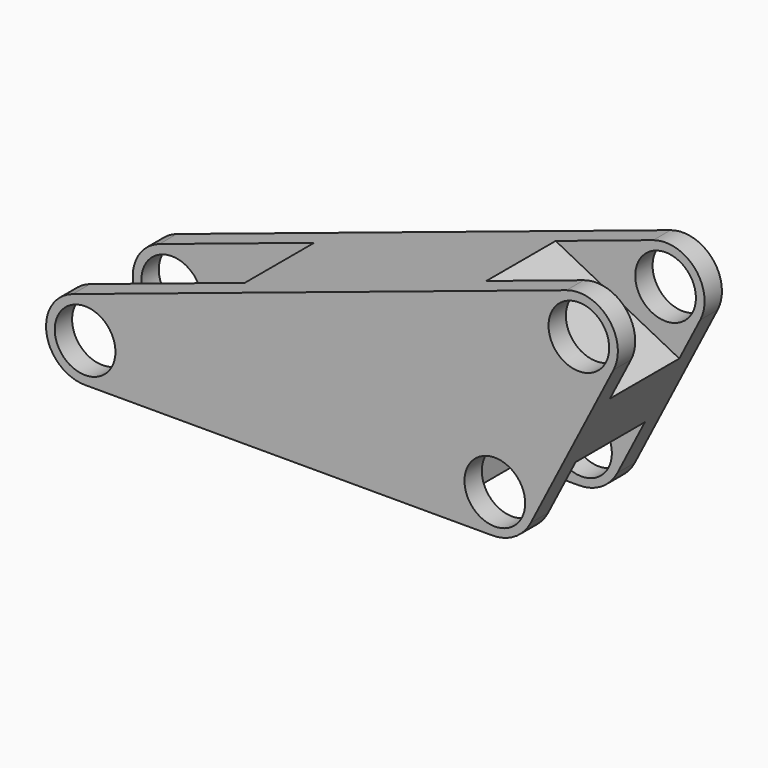
from build123d import *

# Parameters (mm, degrees)
F0_R        = 3.5
F1_DEPTH    = 7.5
F2_W        = 10
F2_H        = 10
F3_DEPTH    = 10
F4_W        = 10
F4_H        = 10
F5_DEPTH    = 10
F6_T1_DEPTH = 10
F7_W        = 10
F7_H        = 14.69305549
F8_DEPTH    = 17.6
F9_DEPTH    = 10
F10_W       = 10
F10_H       = 10
F11_DEPTH   = 25
F12_R       = 5


# Not quite as in the source:
# - a fillet or chamfer that OpenCascade refuses, or shapes differently, is made with other operations: its cross-section is extruded or revolved along the edge and cut away or added
# - a feature of the source that left no trace in its solid (it failed there, or was rolled back) is left out


with BuildPart() as f1:
    # F0 (on Front) → F1 (new body, symmetric)
    with BuildSketch(Plane.XZ):
        with BuildLine():
            ThreePointArc((-12.7951829484, 8.7706469828), (-15.8191748578, 3.7816377734), (-11.3768831394, 0))
            Line((-11.3768831394, 0), (38.6231168606, 0))
            Line((38.6231168606, 0), (49.5697341402, 21.3581733801))
            ThreePointArc((49.5697341402, 21.3581733801), (48.9808970603, 26.3401983487), (44.1467768224, 27.6813111028))
            Line((44.1467768224, 27.6813111028), (-12.7951829484, 8.7706469828))
        make_face()
        with Locations((-11.3768831394, 4.5)):
            Circle(F0_R, mode=Mode.SUBTRACT)
        with Locations((35.8728712662, 4.5)):
            Circle(F0_R, mode=Mode.SUBTRACT)
        with Locations((45.5650766314, 23.41066412)):
            Circle(F0_R, mode=Mode.SUBTRACT)
    extrude(amount=F1_DEPTH, both=True)

    # F2 (on face) → F3 (cut)
    with BuildSketch(Plane(origin=(30.5881386489, 0, -15.6772136421), x_dir=(0, 1, 0), z_dir=(0.8899238908, 0, -0.4561090533))):
        with Locations((0, 22.6163532674)):
            Rectangle(F2_W, F2_H)
    extrude(amount=-F3_DEPTH, mode=Mode.SUBTRACT)

    # F4 (on face) → F5 (cut)
    with BuildSketch(Plane(origin=(0, 0, 0), x_dir=(1, 0, 0), z_dir=(0, 0, -1))):
        with Locations((33.6231168606, 0)):
            Rectangle(F4_W, F4_H)
    extrude(amount=-F5_DEPTH, mode=Mode.SUBTRACT)

    # F6: fillet of radius 19.1889261702 on 1 edges, made by hand

    # F6_s2 → F6_t1 (cut)
    with BuildSketch(Plane.XZ.offset(-5)):
        with BuildLine():
            ThreePointArc((28.6231168606, 10), (31.6047505943, 11.4835737808), (34.2849684854, 13.4603294415))
            Line((34.2849684854, 13.4603294415), (32.5114599843, 10))
            Line((32.5114599843, 10), (28.6231168606, 10))
        make_face()
    extrude(amount=F6_T1_DEPTH, mode=Mode.SUBTRACT)

    # F7 (on Right) → F8 (cut, symmetric)
    with BuildSketch(Plane.YZ):
        with Locations((0, 7.346527745)):
            Rectangle(F7_W, F7_H)
    extrude(amount=F8_DEPTH, both=True, mode=Mode.SUBTRACT)

    # F9 (add): a face of the model
    f9_faces = [f1.faces().sort_by_distance(p)[0] for p in [
        (17.6, 0, 7.346527745),
    ]]
    extrude(f9_faces, amount=F9_DEPTH)

    # F10 (on face) → F11 (cut)
    with BuildSketch(Plane(origin=(30.5881386489, 0, -15.6772136421), x_dir=(0, 1, 0), z_dir=(0.8899238908, 0, -0.4561090533))):
        with Locations((0, 41.310596168)):
            Rectangle(F10_W, F10_H)
    extrude(amount=-F11_DEPTH, mode=Mode.SUBTRACT)

    # F12
    f12_edges = [f1.edges().sort_by_distance(p)[0] for p in [
        (38.623117, 6.25, 0),
        (38.623117, -6.25, 0),
    ]]
    fillet(f12_edges, radius=F12_R)


solid = f1.part
